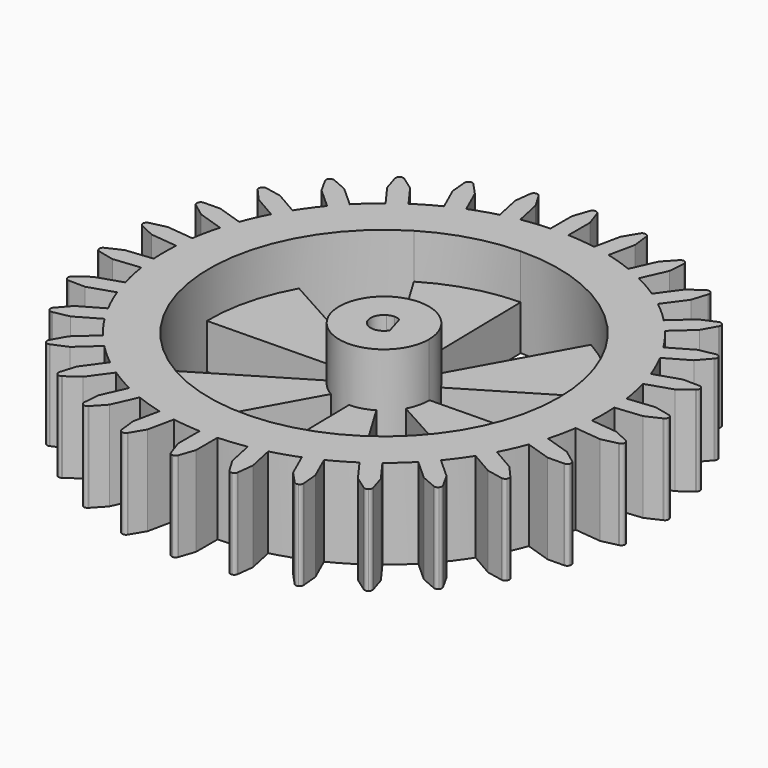
from build123d import *

# Parameters (mm, degrees)
F1_DEPTH        = 20
F2_DEPTH        = 20
F2_COPIES_COUNT = 30
F3_DEPTH        = 10
F3_COPIES_COUNT = 6
F4_DEPTH        = 22


# Not quite as in the source:
# - a pattern or mirror of a feature is missing from the dataset's text; its kind, count and spacing are read off the source's solid


with BuildPart() as f1:
    # F0 (on Top) → F1 (new body)
    with BuildSketch(Plane.XY):
        with BuildLine():
            ThreePointArc((-2, 48.9591666596), (-33.9337590019, -35.3482672843), (49, 0))
            ThreePointArc((49, 0), (35.3482672843, 33.9337590019), (2, 48.9591666596))
            ThreePointArc((2, 48.9591666596), (1.0002083985, 48.9897906013), (0, 49))
            ThreePointArc((0, 49), (-1.0002083985, 48.9897906013), (-2, 48.9591666596))
        make_face()
        with BuildLine():
            ThreePointArc((-0.6771220979, 38.9941214244), (27.3367174162, 27.8155330869), (39, 0))
            ThreePointArc((39, 0), (-19.2060516457, -33.9430048785), (-20.0834656505, 33.4313387029))
            ThreePointArc((-20.0834656505, 33.4313387029), (-10.7464709936, 37.4901768625), (-0.6771220979, 38.9941214244))
        make_face(mode=Mode.SUBTRACT)
    extrude(amount=F1_DEPTH)

    # F0 (on Top) → F2 (join)
    with BuildSketch(Plane.XY):
        with BuildLine():
            ThreePointArc((0, 49), (1.0002083985, 48.9897906013), (2, 48.9591666596))
            Line((2, 48.9591666596), (2, 54.9417920411))
            Line((2, 54.9417920411), (0.8450781533, 58.3315995294))
            Line((0.8450781533, 58.3315995294), (0.7914158491, 58.48910359))
            ThreePointArc((0.7914158491, 58.48910359), (0.4709973959, 58.8611806845), (0, 59))
            Line((0, 59), (0, 49))
        make_face()
        with BuildLine():
            Line((-2, 54.9417920411), (-2, 48.9591666596))
            ThreePointArc((-2, 48.9591666596), (-1.0002083985, 48.9897906013), (0, 49))
            Line((0, 49), (0, 59))
            ThreePointArc((0, 59), (-0.4709973959, 58.8611806845), (-0.7914158491, 58.48910359))
            Line((-0.7914158491, 58.48910359), (-0.8450781533, 58.3315995294))
            Line((-0.8450781533, 58.3315995294), (-2, 54.9417920411))
        make_face()
    f2 = extrude(amount=F2_DEPTH)

    # F2_copies: F2 ×30 about axis
    f2_copies_axis = Axis((0, 0, 0), (0, 0, 1))
    for i in range(1, F2_COPIES_COUNT):
        add(f2.rotate(f2_copies_axis, i * 360 / F2_COPIES_COUNT))

    # F0 (on Top) → F3 (join)
    with BuildSketch(Plane.XY):
        with BuildLine():
            Line((-0.1736210507, 9.9984926729), (-0.6771220979, 38.9941214244))
            ThreePointArc((-0.6771220979, 38.9941214244), (-10.7464709936, 37.4901768625), (-20.0834656505, 33.4313387029))
            Line((-20.0834656505, 33.4313387029), (-5.149606577, 8.5721381289))
            ThreePointArc((-5.149606577, 8.5721381289), (-2.755505383, 9.6128658622), (-0.1736210507, 9.9984926729))
        make_face()
    f3 = extrude(amount=F3_DEPTH)

    # F3_copies: F3 ×6 about axis
    f3_copies_axis = Axis((0, 0, 0), (0, 0, 1))
    for i in range(1, F3_COPIES_COUNT):
        add(f3.rotate(f3_copies_axis, i * 360 / F3_COPIES_COUNT))

    # F0 (on Top) → F4 (join)
    with BuildSketch(Plane.XY):
        with BuildLine():
            ThreePointArc((10, 0), (7.0094147221, 7.132187971), (-0.1736210507, 9.9984926729))
            Line((-0.1736210507, 9.9984926729), (-0.0520863152, 2.9995478019))
            ThreePointArc((-0.0520863152, 2.9995478019), (0.6301122478, 2.9330800458), (1.2794180524, 2.7135013262))
            ThreePointArc((1.2794180524, 2.7135013262), (2.5335996287, 1.606509546), (3, 0))
            ThreePointArc((3, 0), (2.8864879363, -0.8174273019), (2.5545417375, -1.5729960304))
            ThreePointArc((2.5545417375, -1.5729960304), (-2.1329224429, -2.1096544391), (-1.5448819731, 2.5716414387))
            Line((-1.5448819731, 2.5716414387), (-5.149606577, 8.5721381289))
            ThreePointArc((-5.149606577, 8.5721381289), (-4.9246286271, -8.7033345842), (10, 0))
        make_face()
        with BuildLine():
            Line((-0.0520863152, 2.9995478019), (-0.1736210507, 9.9984926729))
            ThreePointArc((-0.1736210507, 9.9984926729), (-2.755505383, 9.6128658622), (-5.149606577, 8.5721381289))
            Line((-5.149606577, 8.5721381289), (-1.5448819731, 2.5716414387))
            ThreePointArc((-1.5448819731, 2.5716414387), (-0.8266516149, 2.8838597587), (-0.0520863152, 2.9995478019))
        make_face()
        with BuildLine():
            ThreePointArc((3, 0), (2.5335996287, 1.606509546), (1.2794180524, 2.7135013262))
            Line((1.2794180524, 2.7135013262), (2.5545417375, -1.5729960304))
            ThreePointArc((2.5545417375, -1.5729960304), (2.8864879363, -0.8174273019), (3, 0))
        make_face()
    extrude(amount=F4_DEPTH)


solid = f1.part
